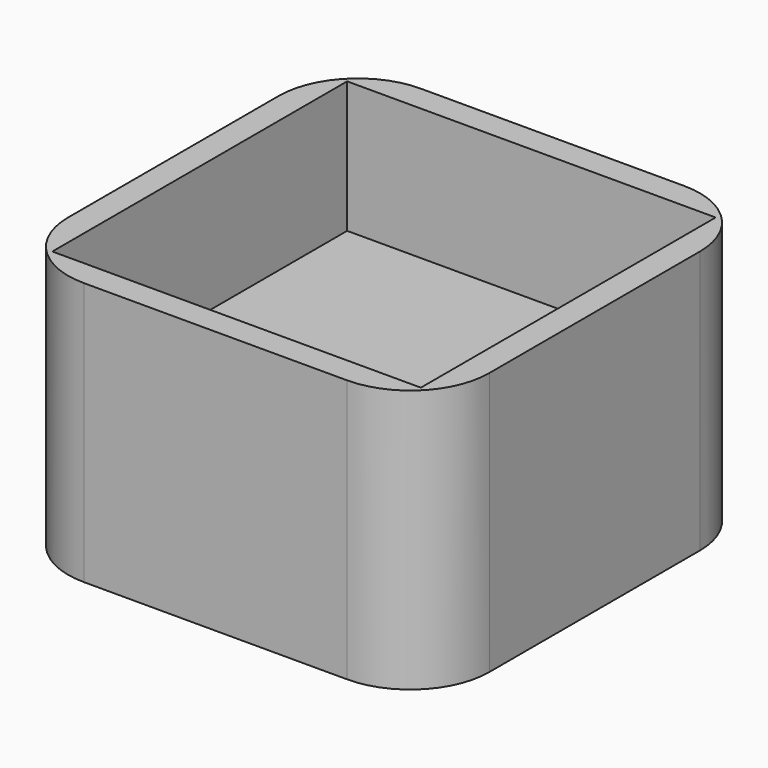
from build123d import *

# Parameters (mm, degrees)
F0_W     = 16
F0_H     = 16
F1_DEPTH = 10
F2_W     = 14
F2_H     = 14
F3_DEPTH = 5
F4_R     = 3


with BuildPart() as f1:
    # F0 (on Top) → F1 (new body)
    with BuildSketch(Plane.XY):
        Rectangle(F0_W, F0_H)
    extrude(amount=F1_DEPTH)

    # F2 (on face) → F3 (cut)
    with BuildSketch(Plane.XY.offset(10)):
        Rectangle(F2_W, F2_H)
    extrude(amount=-F3_DEPTH, mode=Mode.SUBTRACT)

    # F4
    f4_edges = [f1.edges().sort_by_distance(p)[0] for p in [
        (-8, -8, 5),
        (8, -8, 5),
        (8, 8, 5),
        (-8, 8, 5),
    ]]
    fillet(f4_edges, radius=F4_R)


solid = f1.part
